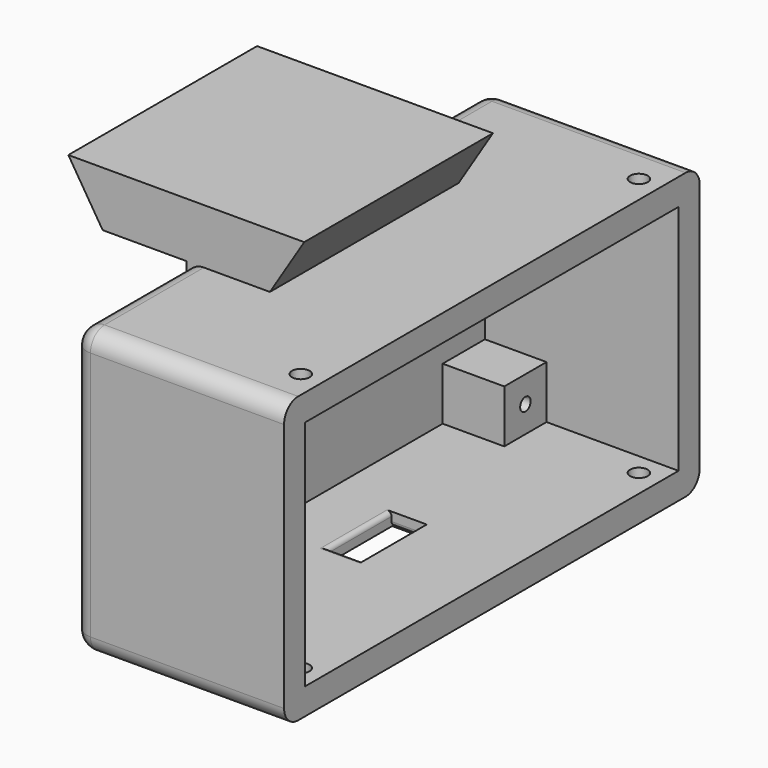
from build123d import *

# Parameters (mm, degrees)
F1_DEPTH  = 26.8
F2_W      = 9.5
F2_H      = 26.8
F3_DEPTH  = 32.4
F4_W      = 53.02
F4_H      = 26.4
F5_DEPTH  = 15
F6_W      = 41.02
F6_H      = 26.4
F7_DEPTH  = 7
F8_W      = 33.1776287834
F8_H      = 14.4
F9_DEPTH  = 7
F10_W     = 16.1501816639
F10_H     = 14.4
F11_DEPTH = 7
F12_R     = 0.6930745825
F13_DEPTH = 5
F14_R     = 0.7453155857
F15_DEPTH = 5
F16_R     = 0.7584591481
F17_DEPTH = 5
F18_R     = 0.7431215043
F19_DEPTH = 5
F20_W     = 4
F20_H     = 9
F21_DEPTH = 5
F22_W     = 10
F22_H     = 13
F23_DEPTH = 1.5
F24_R     = 0.5
F25_R     = 2
F26_R     = 1
F27_DEPTH = 5
F28_R     = 1
F29_DEPTH = 5
F30_R     = 1
F31_DEPTH = 5
F32_R     = 1
F33_DEPTH = 5


with BuildPart() as f1:
    # F0 (on Front) → F1 (new body)
    with BuildSketch(Plane.XZ):
        Polygon((13.4, 0), (-13.4, 0), (-9.5, -6.25), (9.5, -6.25), align=None)
    extrude(amount=F1_DEPTH)

    # F2 (on face) → F3 (join)
    with BuildSketch(Plane(origin=(0, 0, -6.25), x_dir=(1, 0, 0), z_dir=(0, 0, -1))):
        Polygon((24, 42.91), (0, 42.91), (0, 26.8), (9.5, 26.8), (9.5, 0), (0, 0), (0, -16.11), (24, -16.11), align=None)
        with Locations((4.75, 13.4)):
            Rectangle(F2_W, F2_H)
    extrude(amount=F3_DEPTH)

    # F4 (on face) → F5 (cut)
    with BuildSketch(Plane.YZ.offset(24)):
        with Locations((-13.4, -22.45)):
            Rectangle(F4_W, F4_H)
    extrude(amount=-F5_DEPTH, mode=Mode.SUBTRACT)

    # F6 (on face) → F7 (cut)
    with BuildSketch(Plane.YZ.offset(9)):
        with Locations((-13.4, -22.45)):
            Rectangle(F6_W, F6_H)
    extrude(amount=-F7_DEPTH, mode=Mode.SUBTRACT)

    # F8 (on face) → F9 (cut)
    with BuildSketch(Plane.YZ.offset(9)):
        with Locations((-23.3211856083, -22.45)):
            Rectangle(F8_W, F8_H)
    extrude(amount=-F9_DEPTH, mode=Mode.SUBTRACT)

    # F10 (on face) → F11 (cut)
    with BuildSketch(Plane.YZ.offset(9)):
        with Locations((5.0349091681, -22.45)):
            Rectangle(F10_W, F10_H)
    extrude(amount=-F11_DEPTH, mode=Mode.SUBTRACT)

    # F12 (on face) → F13 (cut)
    with BuildSketch(Plane.YZ.offset(9)):
        with Locations((-36.91, -12.25)):
            Circle(F12_R)
    extrude(amount=-F13_DEPTH, mode=Mode.SUBTRACT)

    # F14 (on face) → F15 (cut)
    with BuildSketch(Plane.YZ.offset(9)):
        with Locations((10.11, -12.25)):
            Circle(F14_R)
    extrude(amount=-F15_DEPTH, mode=Mode.SUBTRACT)

    # F16 (on face) → F17 (cut)
    with BuildSketch(Plane.YZ.offset(9)):
        with Locations((-36.91, -32.65)):
            Circle(F16_R)
    extrude(amount=-F17_DEPTH, mode=Mode.SUBTRACT)

    # F18 (on face) → F19 (cut)
    with BuildSketch(Plane.YZ.offset(9)):
        with Locations((10.11, -32.65)):
            Circle(F18_R)
    extrude(amount=-F19_DEPTH, mode=Mode.SUBTRACT)

    # F20 (on face) → F21 (cut)
    with BuildSketch(Plane(origin=(0, 0, -38.65), x_dir=(1, 0, 0), z_dir=(0, 0, -1))):
        with Locations((11, 13.4)):
            Rectangle(F20_W, F20_H)
    extrude(amount=-F21_DEPTH, mode=Mode.SUBTRACT)

    # F22 (on face) → F23 (cut)
    with BuildSketch(Plane(origin=(0, 0, -38.65), x_dir=(1, 0, 0), z_dir=(0, 0, -1))):
        with Locations((10.75, 13.4)):
            Rectangle(F22_W, F22_H)
    extrude(amount=-F23_DEPTH, mode=Mode.SUBTRACT)

    # F24
    f24_edges = [f1.edges().sort_by_distance(p)[0] for p in [
        (5.75, -13.4, -38.65),
        (9, -13.4, -35.65),
        (13, -13.4, -37.15),
        (10.75, -6.9, -38.65),
        (11, -8.9, -37.15),
        (11, -17.9, -35.65),
        (15.75, -13.4, -38.65),
        (10.75, -19.9, -38.65),
    ]]
    fillet(f24_edges, radius=F24_R)

    # F25
    f25_edges = [f1.edges().sort_by_distance(p)[0] for p in [
        (0, -42.91, -22.45),
        (0, -13.4, -38.65),
        (0, 16.11, -22.45),
        (12, -42.91, -38.65),
        (12, -42.91, -6.25),
        (12, 16.11, -38.65),
        (12, 16.11, -6.25),
        (0, 8.055, -6.25),
        (0, -34.855, -6.25),
    ]]
    fillet(f25_edges, radius=F25_R)

    # F26 (on face) → F27 (cut)
    with BuildSketch(Plane(origin=(0, 0, -38.65), x_dir=(1, 0, 0), z_dir=(0, 0, -1))):
        with Locations((21.5, 37.41)):
            Circle(F26_R)
    extrude(amount=-F27_DEPTH, mode=Mode.SUBTRACT)

    # F28 (on face) → F29 (cut)
    with BuildSketch(Plane(origin=(0, 0, -38.65), x_dir=(1, 0, 0), z_dir=(0, 0, -1))):
        with Locations((21.5, -10.61)):
            Circle(F28_R)
    extrude(amount=-F29_DEPTH, mode=Mode.SUBTRACT)

    # F30 (on face) → F31 (cut)
    with BuildSketch(Plane.XY.offset(-6.25)):
        with Locations((21.5, 10.61)):
            Circle(F30_R)
    extrude(amount=-F31_DEPTH, mode=Mode.SUBTRACT)

    # F32 (on face) → F33 (cut)
    with BuildSketch(Plane.XY.offset(-6.25)):
        with Locations((21.5, -37.41)):
            Circle(F32_R)
    extrude(amount=-F33_DEPTH, mode=Mode.SUBTRACT)


solid = f1.part
